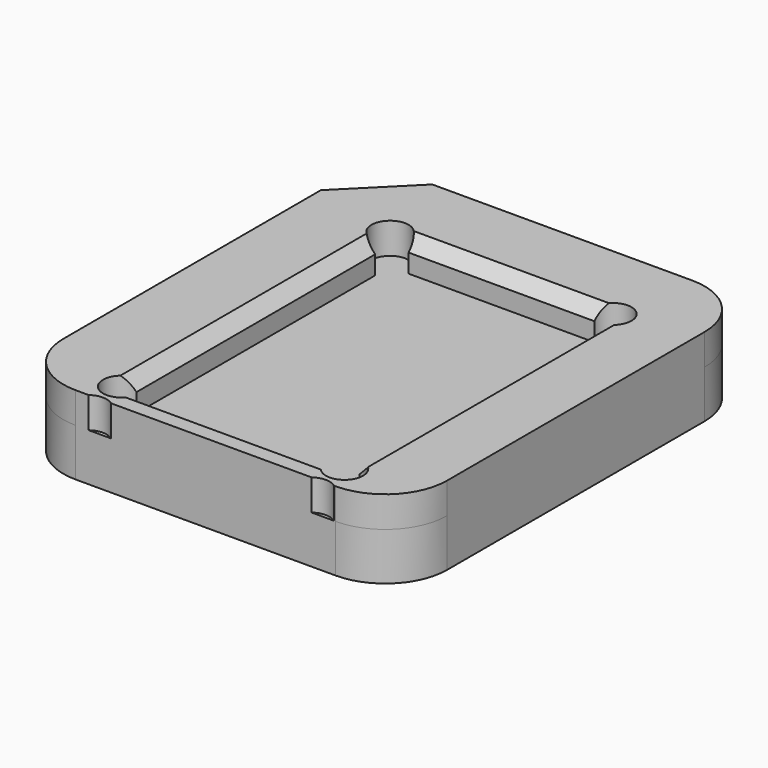
from build123d import *

# Parameters (mm, degrees)
F0_W     = 31
F0_H     = 36
F1_DEPTH = 3.85
F2_SIZE2 = 5
F2_SIZE  = 5
F3_R     = 5
F5_DEPTH = 2.5
F6_SIZE  = 1


with BuildPart() as f1:
    # F0 (on Top) → F1 (new body)
    with BuildSketch(Plane.XY):
        with Locations((15.5, -18)):
            Rectangle(F0_W, F0_H)
    extrude(amount=F1_DEPTH)

    # F2
    f2_edges = [f1.edges().sort_by_distance(p)[0] for p in [
        (0, 0, 1.925),
    ]]
    chamfer(f2_edges, length=F2_SIZE, length2=F2_SIZE2)

    # F3
    f3_edges = [f1.edges().sort_by_distance(p)[0] for p in [
        (31, 0, 1.925),
        (31, -36, 1.925),
        (0, -36, 1.925),
    ]]
    fillet(f3_edges, radius=F3_R)

    # F4 (on face) → F5 (join)
    with BuildSketch(Plane.XY.offset(3.85)):
        with BuildLine():
            Line((5, -36), (6.05, -36))
            ThreePointArc((6.05, -36), (6.95, -35.7), (7.85, -36))
            Line((7.85, -36), (24.05, -36))
            ThreePointArc((24.05, -36), (24.95, -35.7), (25.85, -36))
            Line((25.85, -36), (26, -36))
            ThreePointArc((26, -36), (29.5355339059, -34.5355339059), (31, -31))
            Line((31, -31), (31, -5))
            ThreePointArc((31, -5), (29.5355339059, -1.4644660941), (26, 0))
            Line((26, 0), (5, 0))
            Line((5, 0), (0, -5))
            Line((0, -5), (0, -31))
            ThreePointArc((0, -31), (1.4644660941, -34.5355339059), (5, -36))
        make_face()
        with BuildLine():
            Line((23.45, -33.8), (8.45, -33.8))
            ThreePointArc((8.45, -33.8), (5.8893398282, -34.8606601718), (6.95, -32.3))
            Line((6.95, -32.3), (6.95, -8.2))
            ThreePointArc((6.95, -8.2), (5.8893398282, -5.6393398282), (8.45, -6.7))
            Line((8.45, -6.7), (23.45, -6.7))
            ThreePointArc((23.45, -6.7), (24.95, -5.2), (26.45, -6.7))
            ThreePointArc((26.45, -6.7), (26.0106601718, -7.7606601718), (24.95, -8.2))
            Line((24.95, -8.2), (24.95, -32.3))
            ThreePointArc((24.95, -32.3), (26.0106601718, -32.7393398282), (26.45, -33.8))
            ThreePointArc((26.45, -33.8), (24.95, -35.3), (23.45, -33.8))
        make_face(mode=Mode.SUBTRACT)
    extrude(amount=F5_DEPTH)

    # F6
    f6_edges = [f1.edges().sort_by_distance(p)[0] for p in [
        (6.95, -20.25, 6.35),
        (15.95, -6.7, 6.35),
        (24.95, -20.25, 6.35),
        (15.95, -33.8, 6.35),
    ]]
    chamfer(f6_edges, length=F6_SIZE)


solid = f1.part
